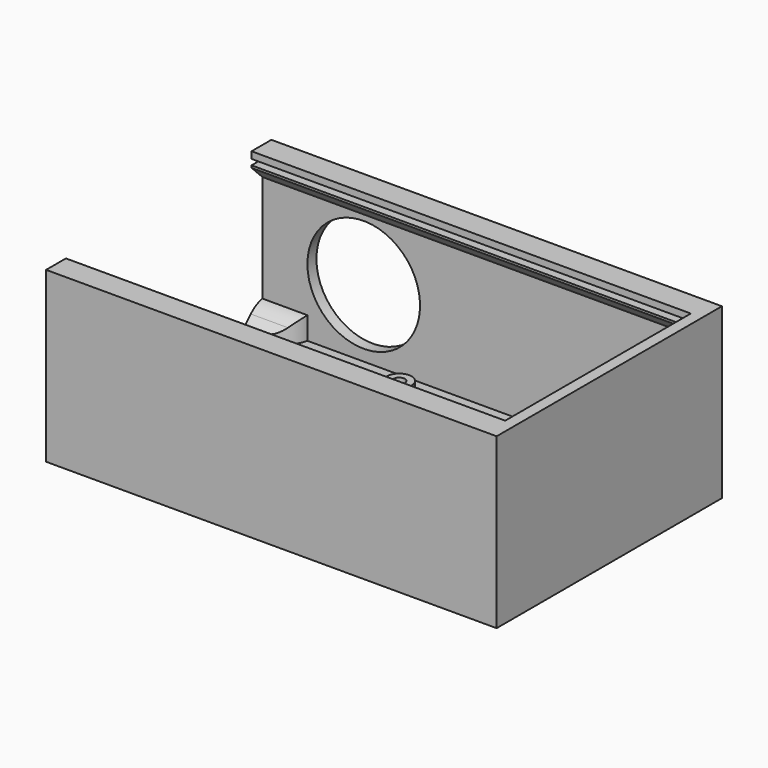
from build123d import *

# Parameters (mm, degrees)
F0_W         = 80
F0_H         = 50
F1_DEPTH     = 30
F2_T         = -2
F3_R         = 2.2
F3_R_2       = 1
F4_DEPTH     = 5.2
F5_W         = 46
F5_H         = 28
F6_DEPTH     = 25
F7_W         = 2.4
F7_H         = 1.2
F8_DEPTH     = 78
F10_DEPTH    = 8
F11_T1_DEPTH = 13.4474487139
F11_T3_DEPTH = 17.690486541
F12_D        = 2
F12_DEPTH    = 6
F12_TIP      = 0.600860619
F14_DEPTH    = 25


# Not quite as in the source:
# - a fillet or chamfer that OpenCascade refuses, or shapes differently, is made with other operations: its cross-section is extruded or revolved along the edge and cut away or added


with BuildPart() as f1:
    # F0 (on Top) → F1 (new body)
    with BuildSketch(Plane.XY):
        Rectangle(F0_W, F0_H)
    extrude(amount=F1_DEPTH)

    # F2
    f2_openings = [f1.faces().sort_by_distance(p)[0] for p in [
        (0, 0, 30),
    ]]
    offset(amount=F2_T, openings=f2_openings)

    # F3 (on face) → F4 (join)
    with BuildSketch(Plane.XY):
        with Locations((-10.7, 16.75)):
            Circle(F3_R)
        with Locations((-10.7, 16.75)):
            Circle(F3_R_2, mode=Mode.SUBTRACT)
        with Locations((-10.7, -16.75)):
            Circle(F3_R)
        with Locations((-10.7, -16.75)):
            Circle(F3_R_2, mode=Mode.SUBTRACT)
        with Locations((33.8, 16.75)):
            Circle(F3_R)
        with Locations((33.8, 16.75)):
            Circle(F3_R_2, mode=Mode.SUBTRACT)
        with Locations((33.8, -16.75)):
            Circle(F3_R)
        with Locations((33.8, -16.75)):
            Circle(F3_R_2, mode=Mode.SUBTRACT)
    extrude(amount=F4_DEPTH)

    # F5 (on face) → F6 (cut)
    with BuildSketch(Plane.YZ.offset(-38)):
        with Locations((0, 16)):
            Rectangle(F5_W, F5_H)
    extrude(amount=-F6_DEPTH, mode=Mode.SUBTRACT)

    # F7 (on face) → F8 (join, through all)
    with BuildSketch(Plane(origin=(-40, 0, 0), x_dir=(0, -1, 0), z_dir=(-1, 0, 0))):
        Polygon((-20.6, 27.8), (-23, 27.8), (-23, 25), (-20.6, 27.4), align=None)
        Polygon((20.6, 26.8), (23, 24.4), (23, 27.8), (20.6, 27.8), align=None)
        with Locations((21.8, 29.4)):
            Rectangle(F7_W, F7_H)
        with Locations((-21.8, 29.4)):
            Rectangle(F7_W, F7_H)
    extrude(amount=-F8_DEPTH)

    # F9 (on face) → F10 (join)
    with BuildSketch(Plane(origin=(-40, 0, 0), x_dir=(0, -1, 0), z_dir=(-1, 0, 0))):
        Polygon((-21.7, 3.3), (-23, 2), (-19, 2), (-19, 3.2), (-20.4, 4.6), align=None)
        Polygon((-23, 6), (-23, 2), (-21.7, 3.3), (-20.4, 4.6), (-21.8, 6), align=None)
        Polygon((19, 2), (23, 2), (23, 6), (21.8, 6), (19, 3.2), align=None)
    extrude(amount=-F10_DEPTH)

    # F11: fillet of radius 5 on 4 edges, made by hand

    # F11_s2 → F11_t1 (cut)
    with BuildSketch(Plane.XY.offset(2)):
        with BuildLine():
            ThreePointArc((-36.8989794856, 19), (-33.7367018254, 20.1270166538), (-32, 23))
            Line((-32, 23), (-32, 19))
            Line((-32, 19), (-36.8989794856, 19))
        make_face()
        with BuildLine():
            ThreePointArc((-36.8989794856, -19), (-33.7367018254, -20.1270166538), (-32, -23))
            Line((-32, -23), (-32, -19))
            Line((-32, -19), (-36.8989794856, -19))
        make_face()
    extrude(amount=F11_T1_DEPTH, mode=Mode.SUBTRACT)

    # F11_s4 → F11_t3 (cut)
    with BuildSketch(Plane.YZ.offset(-44.8452432705)):
        with BuildLine():
            ThreePointArc((-23, 6), (-21.6127664169, 5.5061172285), (-20.4295582508, 4.6295582508))
            Line((-20.4295582508, 4.6295582508), (-21.8, 6))
            Line((-21.8, 6), (-23, 6))
        make_face()
        with BuildLine():
            ThreePointArc((20.4295582508, 4.6295582508), (21.6127664169, 5.5061172285), (23, 6))
            Line((23, 6), (21.8, 6))
            Line((21.8, 6), (20.4295582508, 4.6295582508))
        make_face()
    extrude(amount=F11_T3_DEPTH, mode=Mode.SUBTRACT)

    # F12
    with Locations(Plane(origin=(-40, 0, 0), x_dir=(0, -1, 0), z_dir=(-1, 0, 0))):
        with Locations((-21.7, 3.3), (21.7, 3.3)):
            Hole(F12_D / 2, depth=F12_DEPTH)
            with Locations((0, 0, -(F12_DEPTH + F12_TIP / 2))):  # 118° drill point
                Cone(0, F12_D / 2, F12_TIP, mode=Mode.SUBTRACT)

    # F13 (on face) → F14 (cut)
    with BuildSketch(Plane.XZ.offset(-23)):
        with BuildLine():
            ThreePointArc((-28, 6), (-17.527864045, 5.05572809), (-12, 14))
            ThreePointArc((-12, 14), (-22, 24), (-32, 14))
            ThreePointArc((-32, 14), (-30.94427191, 9.527864045), (-28, 6))
        make_face()
        with BuildLine():
            ThreePointArc((30, 21.8), (25.2, 17), (30, 12.2))
            Line((30, 12.2), (30, 17))
            Line((30, 17), (30, 21.8))
        make_face()
        with BuildLine():
            ThreePointArc((34.8, 17), (33.3941125497, 20.3941125497), (30, 21.8))
            Line((30, 21.8), (30, 17))
            Line((30, 17), (34.8, 17))
        make_face()
        with BuildLine():
            Line((30, 17), (30, 12.2))
            ThreePointArc((30, 12.2), (33.3941125497, 13.6058874503), (34.8, 17))
            Line((34.8, 17), (30, 17))
        make_face()
    extrude(amount=-F14_DEPTH, mode=Mode.SUBTRACT)


solid = f1.part
